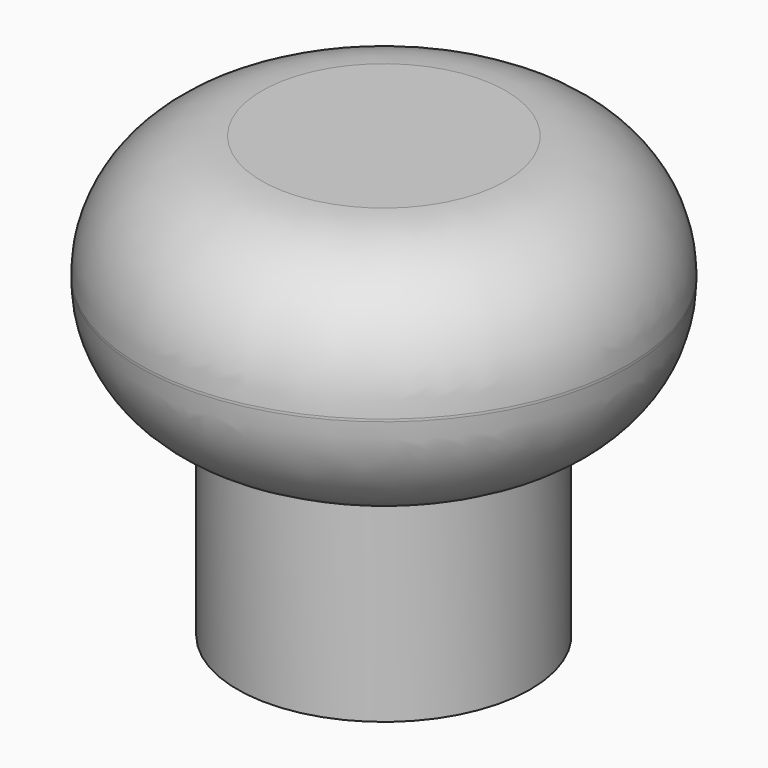
from build123d import *

# Parameters (mm, degrees)
F0_R     = 15
F1_DEPTH = 20
F2_R     = 25
F3_DEPTH = 25


# Not quite as in the source:
# - a fillet or chamfer that OpenCascade refuses, or shapes differently, is made with other operations: its cross-section is extruded or revolved along the edge and cut away or added


with BuildPart() as f1:
    # F0 (on Top) → F1 (new body)
    with BuildSketch(Plane.XY):
        Circle(F0_R)
    extrude(amount=F1_DEPTH)

    # F2 (on face) → F3 (join)
    with BuildSketch(Plane.XY.offset(20)):
        Circle(F2_R)
    extrude(amount=F3_DEPTH)

    # F4: fillet of radius 12.5 on 2 edges, made by hand

    # F4_s1 → F4_t2 (revolve, cut)
    with BuildSketch(Plane.XZ):
        with BuildLine():
            ThreePointArc((25, 32.5), (21.3388347648, 41.3388347648), (12.5, 45))
            Line((12.5, 45), (25, 45))
            Line((25, 45), (25, 32.5))
        make_face()
    revolve(axis=Axis((0, 0, 45), (0, 0, 1)), mode=Mode.SUBTRACT)

    # F4_s3 → F4_t4 (revolve, cut)
    with BuildSketch(Plane.XZ):
        with BuildLine():
            ThreePointArc((25, 32.2474487139), (22.1824583655, 24.3417545635), (15, 20))
            Line((15, 20), (25, 20))
            Line((25, 20), (25, 32.2474487139))
        make_face()
    revolve(axis=Axis((0, 0, 20), (0, 0, 1)), mode=Mode.SUBTRACT)


solid = f1.part
